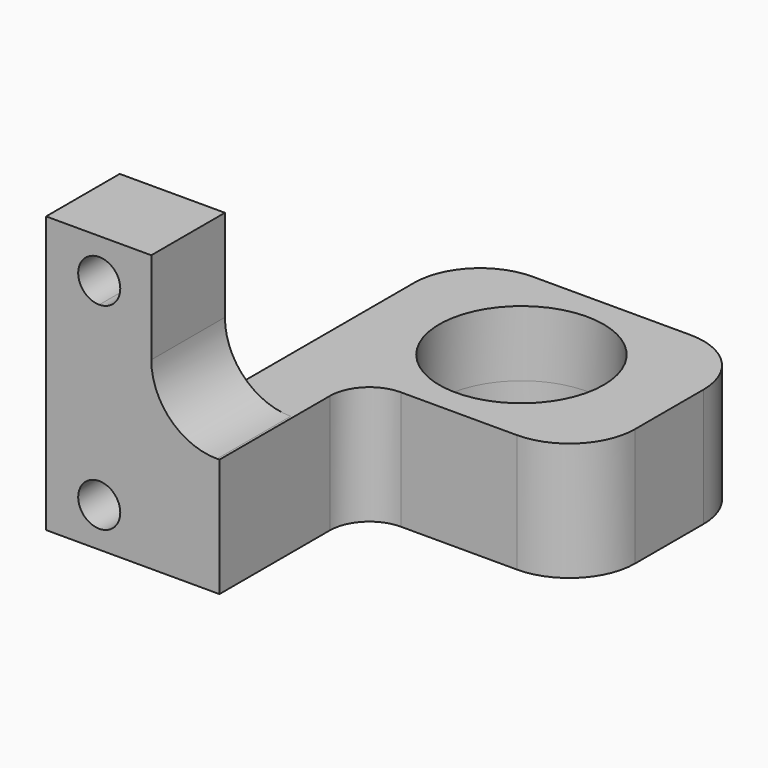
from build123d import *

# Parameters (mm, degrees)
F0_W      = 28
F0_H      = 30
F1_DEPTH  = 4
F2_R      = 6.25
F2_W      = 6
F2_H      = 23
F2_W_2    = 16.817460835
F2_H_2    = 13.5
F3_DEPTH  = 25
F4_W      = 6
F4_H      = 7
F4_R      = 6.25
F5_DEPTH  = 5
F6_DEPTH  = 17
F8_DEPTH  = 25
F9_R      = 5
F10_R     = 3
F11_R     = 5
F12_DEPTH = 2


with BuildPart() as f1:
    # F0 (on Top) → F1 (new body)
    with BuildSketch(Plane.XY):
        with Locations((14, 15)):
            Rectangle(F0_W, F0_H)
    extrude(amount=F1_DEPTH)

    # F2 (on face) → F3 (cut)
    with BuildSketch(Plane.XY.offset(4)):
        with Locations((16.75, 21.75)):
            Circle(F2_R)
        with Locations((3, 18.5)):
            Rectangle(F2_W, F2_H)
        with Locations((19.5912695825, 6.75)):
            Rectangle(F2_W_2, F2_H_2)
    extrude(amount=-F3_DEPTH, mode=Mode.SUBTRACT)

    # F4 (on face) → F5 (join)
    with BuildSketch(Plane.XY.offset(4)):
        with Locations((3, 3.5)):
            Rectangle(F4_W, F4_H)
        Polygon((6, 30), (6, 7), (6, 0), (11.182539165, 0), (11.182539165, 13.5), (28, 13.5), (28, 30), align=None)
        with Locations((16.75, 21.75)):
            Circle(F4_R, mode=Mode.SUBTRACT)
    extrude(amount=F5_DEPTH)

    # F4 (on face) → F6 (join)
    with BuildSketch(Plane.XY.offset(4)):
        with Locations((3, 3.5)):
            Rectangle(F4_W, F4_H)
    extrude(amount=F6_DEPTH)

    # F7 (on face) → F8 (cut)
    with BuildSketch(Plane.XZ):
        with BuildLine():
            ThreePointArc((3.6420098484, 3), (3.1733806983, 4.1313708499), (2.0420098484, 4.6))
            ThreePointArc((2.0420098484, 4.6), (0.9106389985, 1.8686291501), (3.6420098484, 3))
        make_face()
        with BuildLine():
            ThreePointArc((3.6420098484, 18), (0.9106389985, 19.1313708499), (2.0420098484, 16.4))
            ThreePointArc((2.0420098484, 16.4), (3.1733806983, 16.8686291501), (3.6420098484, 18))
        make_face()
    extrude(amount=-F8_DEPTH, mode=Mode.SUBTRACT)

    # F9
    f9_edges = [f1.edges().sort_by_distance(p)[0] for p in [
        (28, 13.5, 4.5),
        (28, 30, 4.5),
        (6, 30, 4.5),
    ]]
    fillet(f9_edges, radius=F9_R)

    # F10
    f10_edges = [f1.edges().sort_by_distance(p)[0] for p in [
        (11.182539, 13.5, 4.5),
    ]]
    fillet(f10_edges, radius=F10_R)

    # F11
    f11_edges = [f1.edges().sort_by_distance(p)[0] for p in [
        (6, 3.5, 9),
    ]]
    fillet(f11_edges, radius=F11_R)

    # F12 (add): a face of the model
    f12_faces = [f1.faces().sort_by_distance(p)[0] for p in [
        (0, 3.5, 10.5),
    ]]
    extrude(f12_faces, amount=F12_DEPTH)


solid = f1.part
